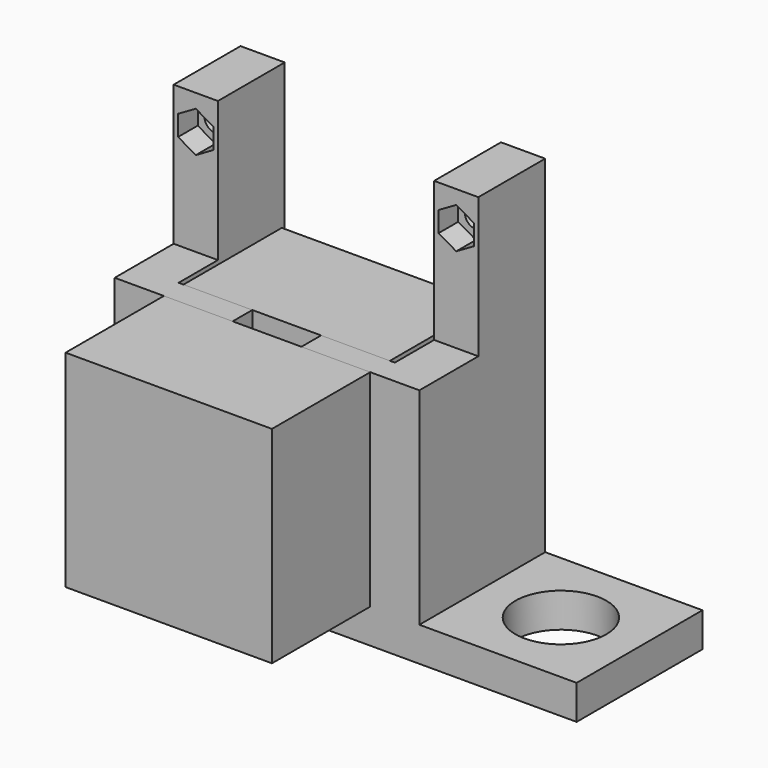
from build123d import *

# Parameters (mm, degrees)
F1_R      = 2.25
F2_DEPTH  = 12
F4_DEPTH  = 5
F5_W      = 44
F5_H      = 10
F5_H_2    = 5
F6_DEPTH  = 7
F7_DEPTH  = 42
F8_R      = 1.7
F8_R_2    = 13
F9_DEPTH  = 5
F11_REACH = 63.8670687473
F12_R     = 1.7
F13_DEPTH = 25
F14_W     = 42
F14_H     = 42
F14_R     = 1.7
F14_R_2   = 13
F15_DEPTH = 25
F16_W     = 32
F16_H     = 32
F16_R     = 9.25
F17_DEPTH = 7


with BuildPart() as f2:
    # F1 (on Front) → F2 (new body)
    with BuildSketch(Plane.XZ):
        Polygon((-27, 56.5), (-36, 56.5), (-36, -21), (26, -21), (26, 56.5), (17, 56.5), (17, -14), (-27, -14), align=None)
        with Locations((-31.5, 49.5)):
            Circle(F1_R, mode=Mode.SUBTRACT)
        with Locations((21.5, 49.5)):
            Circle(F1_R, mode=Mode.SUBTRACT)
    extrude(amount=-F2_DEPTH)

    # F3 (on face) → F4 (join)
    with BuildSketch(Plane.XZ):
        Polygon((-27, -14), (-27, 56.5), (-36, 56.5), (-36, -21), (26, -21), (26, 56.5), (17, 56.5), (17, -14), align=None)
        Polygon((-31.5, 53.6569219382), (-27.9, 51.5784609691), (-27.9, 47.4215390309), (-31.5, 45.3430780618), (-35.1, 47.4215390309), (-35.1, 51.5784609691), align=None, mode=Mode.SUBTRACT)
        Polygon((21.5, 53.6569219382), (25.1, 51.5784609691), (25.1, 47.4215390309), (21.5, 45.3430780618), (17.9, 47.4215390309), (17.9, 51.5784609691), align=None, mode=Mode.SUBTRACT)
    extrude(amount=F4_DEPTH)

    # F5 (on face) → F6 (join, through all)
    with BuildSketch(Plane.XY.offset(-14)):
        with Locations((-5, -10)):
            Rectangle(F5_W, F5_H)
        with Locations((-5, -17.5)):
            Rectangle(F5_W, F5_H_2)
        Polygon((-27, -15), (-27, -5), (-36, -5), (-36, -20), (-27, -20), align=None)
        Polygon((26, -5), (17, -5), (17, -15), (17, -20), (26, -20), align=None)
    extrude(amount=-F6_DEPTH)

    # F5 (on face) → F7 (join)
    with BuildSketch(Plane.XY.offset(-14)):
        with Locations((-5, -17.5)):
            Rectangle(F5_W, F5_H_2)
        Polygon((-27, -15), (-27, -5), (-36, -5), (-36, -20), (-27, -20), align=None)
        Polygon((26, -5), (17, -5), (17, -15), (17, -20), (26, -20), align=None)
    extrude(amount=F7_DEPTH)

    # F8 (on face) → F9 (cut, through all)
    with BuildSketch(Plane.XZ.offset(20)):
        with Locations((-20.5, 22.5)):
            Circle(F8_R)
        with Locations((-5, 7)):
            Circle(F8_R_2)
        with Locations((-20.5, -8.5)):
            Circle(F8_R)
        with Locations((10.5, -8.5)):
            Circle(F8_R)
        with Locations((10.5, 22.5)):
            Circle(F8_R)
    extrude(amount=-F9_DEPTH, mode=Mode.SUBTRACT)

    f11_end = f2.faces().sort_by_distance((-18, -17.5, 7))[0]
    # F10 (on face) → F11 (cut, up to a face of the model that its end follows)
    with BuildSketch(Plane.XY.offset(28)):
        Polygon((2, -15), (-5, -15), (-12, -15), (-12, -20), (2, -20), align=None)
    f11_long = extrude(amount=-F11_REACH, mode=Mode.PRIVATE)
    add(split(f11_long, bisect_by=f11_end, keep=Keep.ALL, mode=Mode.PRIVATE).solids().sort_by_distance((-5, -17.5, 28))[0], mode=Mode.SUBTRACT)

    # F16 (on face) → F17 (join, through all)
    with BuildSketch(Plane(origin=(0, 0, -21), x_dir=(1, 0, 0), z_dir=(0, 0, -1))):
        with Locations((42, 4)):
            Rectangle(F16_W, F16_H)
        with Locations((42, 4)):
            Circle(F16_R, mode=Mode.SUBTRACT)
    extrude(amount=-F17_DEPTH)


with BuildPart() as f13:
    # F12 (on face) → F13 (new body)
    with BuildSketch(Plane(origin=(0, -15, 0), x_dir=(-1, 0, 0), z_dir=(0, 1, 0))):
        with BuildLine():
            Line((-16, -14), (26, -14))
            Line((26, -14), (26, 28))
            Line((26, 28), (12, 28))
            Line((12, 28), (12, 17.9544511501))
            ThreePointArc((12, 17.9544511501), (5, -6), (-2, 17.9544511501))
            Line((-2, 17.9544511501), (-2, 28))
            Line((-2, 28), (-16, 28))
            Line((-16, 28), (-16, -14))
        make_face()
        with Locations((-10.5, -8.5)):
            Circle(F12_R, mode=Mode.SUBTRACT)
        with Locations((20.5, -8.5)):
            Circle(F12_R, mode=Mode.SUBTRACT)
        with Locations((-10.5, 22.5)):
            Circle(F12_R, mode=Mode.SUBTRACT)
        with Locations((20.5, 22.5)):
            Circle(F12_R, mode=Mode.SUBTRACT)
        with BuildLine():
            Line((12, 17.9544511501), (12, 28))
            Line((12, 28), (-2, 28))
            Line((-2, 28), (-2, 17.9544511501))
            ThreePointArc((-2, 17.9544511501), (5, -6), (12, 17.9544511501))
        make_face()
        with Locations((-10.5, 22.5)):
            Circle(F12_R)
        with Locations((20.5, 22.5)):
            Circle(F12_R)
        with Locations((-10.5, -8.5)):
            Circle(F12_R)
        with Locations((20.5, -8.5)):
            Circle(F12_R)
    extrude(amount=F13_DEPTH)


with BuildPart() as f15:
    # F14 (on face) → F15 (new body)
    with BuildSketch(Plane.XZ.offset(20)):
        with Locations((-5, 7)):
            Rectangle(F14_W, F14_H)
        with Locations((-20.5, -8.5)):
            Circle(F14_R, mode=Mode.SUBTRACT)
        with Locations((10.5, -8.5)):
            Circle(F14_R, mode=Mode.SUBTRACT)
        with Locations((-20.5, 22.5)):
            Circle(F14_R, mode=Mode.SUBTRACT)
        with Locations((-5, 7)):
            Circle(F14_R_2, mode=Mode.SUBTRACT)
        with Locations((10.5, 22.5)):
            Circle(F14_R, mode=Mode.SUBTRACT)
    extrude(amount=F15_DEPTH)

    # F8 (on face) → F15, piece 2 (join)
    with BuildSketch(Plane.XZ.offset(20)):
        with Locations((-20.5, 22.5)):
            Circle(F8_R)
    extrude(amount=F15_DEPTH)

    # F8 (on face) → F15, piece 3 (join)
    with BuildSketch(Plane.XZ.offset(20)):
        with Locations((-5, 7)):
            Circle(F8_R_2)
    extrude(amount=F15_DEPTH)

    # F8 (on face) → F15, piece 4 (join)
    with BuildSketch(Plane.XZ.offset(20)):
        with Locations((-20.5, -8.5)):
            Circle(F8_R)
    extrude(amount=F15_DEPTH)

    # F8 (on face) → F15, piece 5 (join)
    with BuildSketch(Plane.XZ.offset(20)):
        with Locations((10.5, 22.5)):
            Circle(F8_R)
    extrude(amount=F15_DEPTH)

    # F8 (on face) → F15, piece 6 (join)
    with BuildSketch(Plane.XZ.offset(20)):
        with Locations((10.5, -8.5)):
            Circle(F8_R)
    extrude(amount=F15_DEPTH)


solid = Compound([f2.part, f13.part, f15.part])
